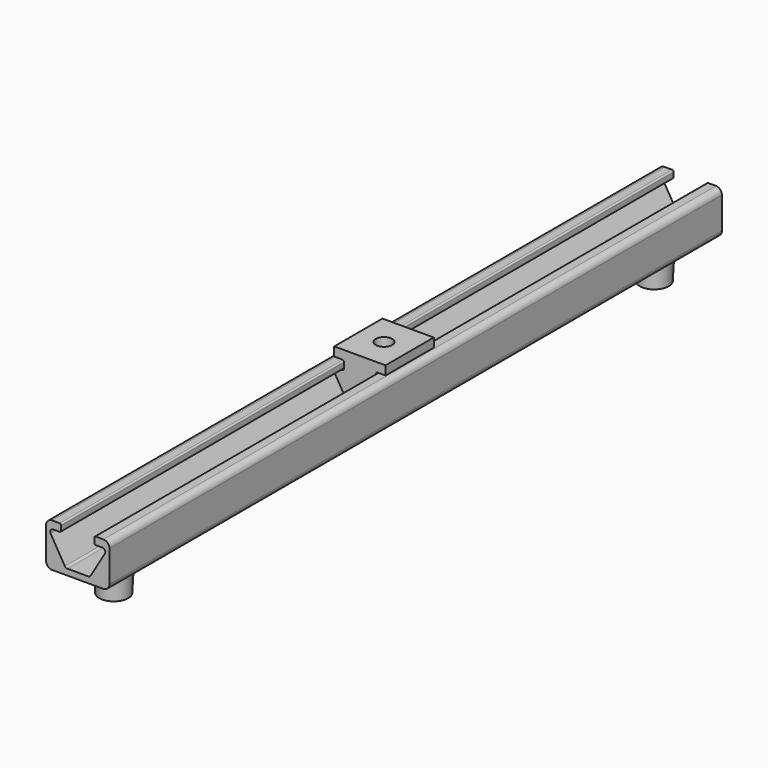
from build123d import *

# Parameters (mm, degrees)
F1_DEPTH = 127
F3_DEPTH = 10
F5_D     = 5.5
F5_DEPTH = 90
F5_TIP   = 1.6523667023
F6_R     = 5.3298784099
F7_DEPTH = 10
F7_TAPER = 3


# Not quite as in the source:
# - a pattern or mirror of a feature is missing from the dataset's text; its kind, count and spacing are read off the source's solid


with BuildPart() as f1:
    # F0 (on Front) → F1 (new body, symmetric)
    with BuildSketch(Plane.XZ):
        with BuildLine():
            ThreePointArc((10.5092503586, 5.2297932934), (9.923463921, 6.6440068557), (8.5092503586, 7.2297932934))
            Line((8.5092503586, 7.2297932934), (5.9933694905, 7.2297932934))
            ThreePointArc((5.9933694905, 7.2297932934), (5.6398160999, 7.083346684), (5.4933694905, 6.7297932934))
            Line((5.4933694905, 6.7297932934), (5.4933694905, 5.2297932934))
            ThreePointArc((5.4933694905, 5.2297932934), (5.6398160999, 4.8762399028), (5.9933694905, 4.7297932934))
            Line((5.9933694905, 4.7297932934), (8.1368030805, 4.7297932934))
            ThreePointArc((8.1368030805, 4.7297932934), (9.0055991387, 4.2249633746), (8.9972067099, 3.220180112))
            Line((8.9972067099, 3.220180112), (4.2904538965, -4.726449511))
            ThreePointArc((4.2904538965, -4.726449511), (3.9252203484, -5.0856323878), (3.4300502672, -5.2168363297))
            Line((3.4300502672, -5.2168363297), (0, -5.2168363297))
            Line((0, -5.2168363297), (-3.4300502672, -5.2168363297))
            ThreePointArc((-3.4300502672, -5.2168363297), (-3.9252203484, -5.0856323878), (-4.2904538965, -4.726449511))
            Line((-4.2904538965, -4.726449511), (-8.9972067099, 3.220180112))
            ThreePointArc((-8.9972067099, 3.220180112), (-9.0055991387, 4.2249633746), (-8.1368030805, 4.7297932934))
            Line((-8.1368030805, 4.7297932934), (-5.9933694905, 4.7297932934))
            ThreePointArc((-5.9933694905, 4.7297932934), (-5.6398160999, 4.8762399028), (-5.4933694905, 5.2297932934))
            Line((-5.4933694905, 5.2297932934), (-5.4933694905, 6.7297932934))
            ThreePointArc((-5.4933694905, 6.7297932934), (-5.6398160999, 7.083346684), (-5.9933694905, 7.2297932934))
            Line((-5.9933694905, 7.2297932934), (-8.5092503586, 7.2297932934))
            ThreePointArc((-8.5092503586, 7.2297932934), (-9.923463921, 6.6440068557), (-10.5092503586, 5.2297932934))
            Line((-10.5092503586, 5.2297932934), (-10.5092503586, -5.2297932934))
            ThreePointArc((-10.5092503586, -5.2297932934), (-9.923463921, -6.6440068557), (-8.5092503586, -7.2297932934))
            Line((-8.5092503586, -7.2297932934), (8.5092503586, -7.2297932934))
            ThreePointArc((8.5092503586, -7.2297932934), (9.923463921, -6.6440068557), (10.5092503586, -5.2297932934))
            Line((10.5092503586, -5.2297932934), (10.5092503586, 5.2297932934))
        make_face()
    extrude(amount=F1_DEPTH, both=True)

    # F6 (on face) → F7 (join)
    with BuildSketch(Plane(origin=(0, 0, -7.2297932934), x_dir=(1, 0, 0), z_dir=(0, 0, -1))):
        with Locations((0, -112.07459867)):
            Circle(F6_R)
    f7 = extrude(amount=F7_DEPTH, taper=F7_TAPER)

    # F7_copies: F7 across plane
    add(f7.mirror(Plane(origin=(0, 0, 0), x_dir=(0, 0, -1), z_dir=(0, -1, 0))))


with BuildPart() as f3:
    # F2 (on Front) → F3 (new body, symmetric)
    with BuildSketch(Plane.XZ):
        with BuildLine():
            Line((5.9933694905, 7.5297932934), (8.5092503586, 7.5297932934))
            Line((8.5092503586, 7.5297932934), (8.5092503586, 10.502230376))
            Line((8.5092503586, 10.502230376), (-8.5092503586, 10.502230376))
            Line((-8.5092503586, 10.502230376), (-8.5092503586, 7.5297932934))
            Line((-8.5092503586, 7.5297932934), (-5.9933694905, 7.5297932934))
            ThreePointArc((-5.9933694905, 7.5297932934), (-5.4276840655, 7.2954787183), (-5.1933694905, 6.7297932934))
            Line((-5.1933694905, 6.7297932934), (-5.1933694905, 5.2297932934))
            ThreePointArc((-5.1933694905, 5.2297932934), (-5.4276840655, 4.6641078684), (-5.9933694905, 4.4297932934))
            Line((-5.9933694905, 4.4297932934), (-8.1368030805, 4.4297932934))
            ThreePointArc((-8.1368030805, 4.4297932934), (-8.7449603212, 4.0764123502), (-8.7390856211, 3.3730640664))
            Line((-8.7390856211, 3.3730640664), (-4.0323328077, -4.5735655566))
            ThreePointArc((-4.0323328077, -4.5735655566), (-3.776669324, -4.8249935704), (-3.4300502672, -4.9168363297))
            Line((-3.4300502672, -4.9168363297), (3.4300502672, -4.9168363297))
            ThreePointArc((3.4300502672, -4.9168363859), (3.7766693519, -4.8249936193), (4.0323328561, -4.5735655853))
            Line((4.0323328077, -4.5735655566), (8.7390856211, 3.3730640664))
            ThreePointArc((8.7390856211, 3.3730640664), (8.7449603212, 4.0764123502), (8.1368030805, 4.4297932934))
            Line((8.1368030805, 4.4297932934), (5.9933694905, 4.4297932934))
            ThreePointArc((5.9933694905, 4.4297932934), (5.4276840655, 4.6641078684), (5.1933694905, 5.2297932934))
            Line((5.1933694905, 5.2297932934), (5.1933694905, 6.7297932934))
            ThreePointArc((5.1933694905, 6.7297932934), (5.4276840655, 7.2954787183), (5.9933694905, 7.5297932934))
        make_face()
    extrude(amount=F3_DEPTH, both=True)

    # F5
    with Locations(Plane.XY.offset(10.502230376)):
        with Locations((0, 0)):
            Hole(F5_D / 2, depth=F5_DEPTH)
            with Locations((0, 0, -(F5_DEPTH + F5_TIP / 2))):  # 118° drill point
                Cone(0, F5_D / 2, F5_TIP, mode=Mode.SUBTRACT)


solid = Compound([f1.part, f3.part])
